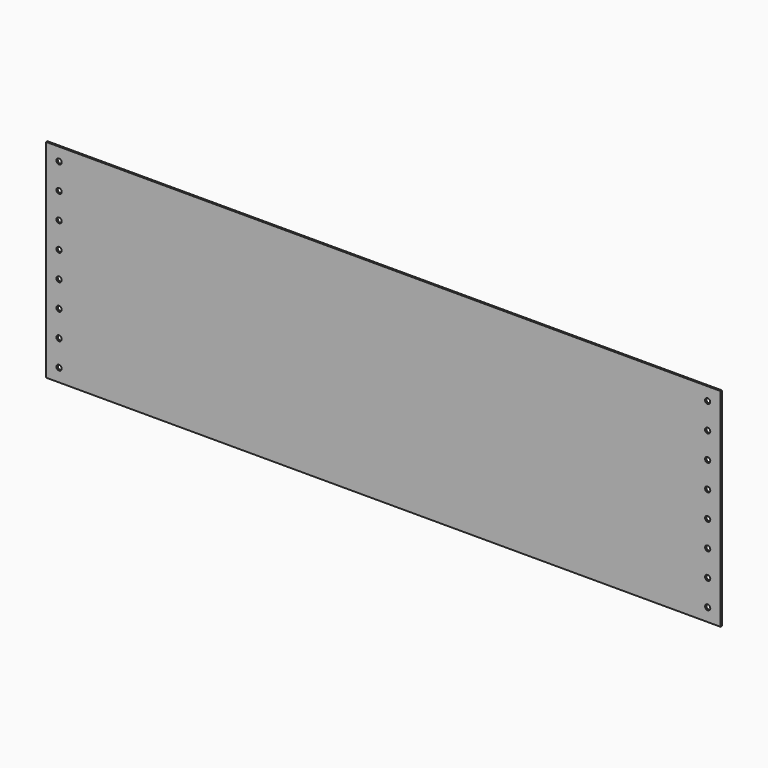
from build123d import *

# Parameters (mm, degrees)
F0_W     = 660.4
F0_H     = 203.2
F1_DEPTH = 1.5875
F3_D     = 5.1054


# Not quite as in the source:
# - a length typed as a fraction of an inch, garbled in the dataset ("3 / 203.2 mm" for 3/8 in), is restored


with BuildPart() as f1:
    # F0 (on Front) → F1 (new body)
    with BuildSketch(Plane.XZ):
        with Locations((1.7192233354, -130.3142405412)):
            Rectangle(F0_W, F0_H)
    extrude(amount=F1_DEPTH)

    # F3 (through all)
    with Locations(Plane.XZ.offset(1.5875)):
        with Locations((-315.7807766646, -92.2142405412), (-315.7807766646, -117.6142405412), (-315.7807766646, -143.0142405412), (319.2192233354, -219.2142405412), (319.2192233354, -168.4142405412), (319.2192233354, -117.6142405412), (319.2192233354, -66.8142405412), (319.2192233354, -193.8142405412), (319.2192233354, -143.0142405412), (-315.7807766646, -168.4142405412), (319.2192233354, -92.2142405412), (-315.7807766646, -193.8142405412), (-315.7807766646, -219.2142405412), (-315.7807766646, -41.4142405412), (-315.7807766646, -66.8142405412), (319.2192233354, -41.4142405412)):
            Hole(F3_D / 2)


solid = f1.part
